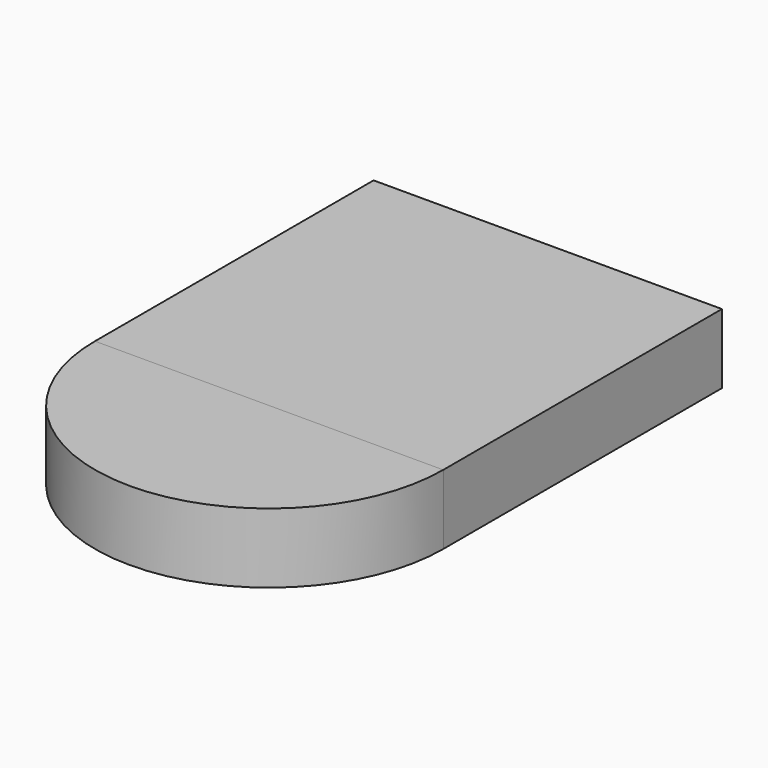
from build123d import *

# Parameters (mm, degrees)
F0_W     = 1524
F0_H     = 1524
F1_DEPTH = 304.8
F3_DEPTH = 304.8


# Not quite as in the source:
# - a feature of the source that left no trace in its solid (it failed there, or was rolled back) is left out


with BuildPart() as f1:
    # F0 (on Top) → F1 (new body)
    with BuildSketch(Plane.XY):
        with Locations((762, -762)):
            Rectangle(F0_W, F0_H)
    extrude(amount=F1_DEPTH)


with BuildPart() as f3:
    # F2 (on face) → F3 (new body)
    with BuildSketch(Plane.XY.offset(304.8)):
        with BuildLine():
            ThreePointArc((0, -1524), (762, -2286), (1524, -1524))
            Line((1524, -1524), (0, -1524))
        make_face()
    extrude(amount=-F3_DEPTH)


solid = Compound([f1.part, f3.part])
